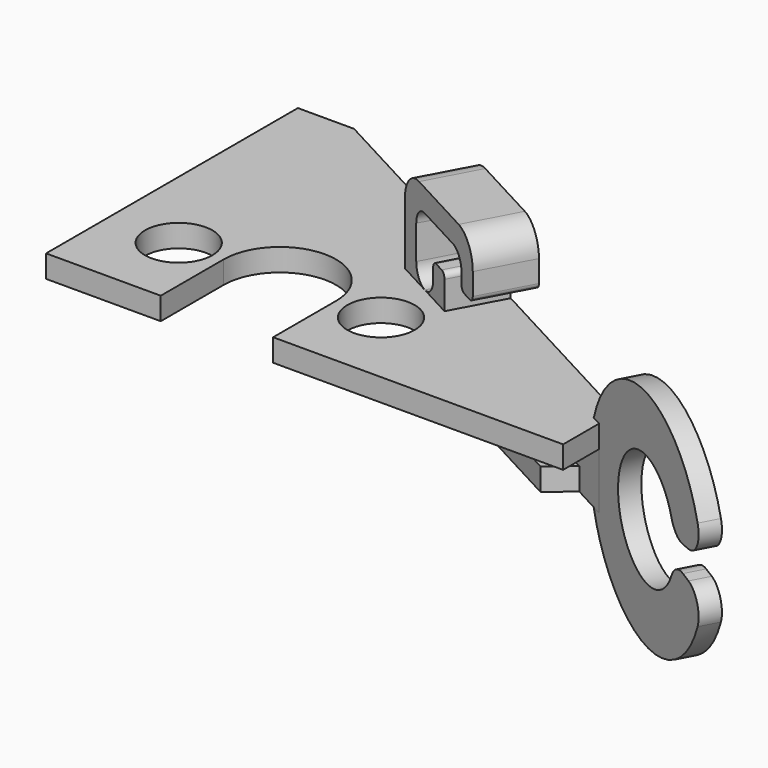
from build123d import *

# Parameters (mm, degrees)
F1_DEPTH  = 2
F2_R      = 3
F3_DEPTH  = 2
F4_W      = 2
F4_H      = 3
F5_DEPTH  = 5
F6_R      = 2.5
F7_R      = 1.49999
F8_R      = 0.5
F10_DEPTH = 5
F12_DEPTH = 2
F13_R     = 9.9401429079
F13_R_2   = 5
F14_DEPTH = 1.7623205361
F16_DEPTH = 1.7623205361
F17_R     = 2


# Not quite as in the source:
# - a fillet or chamfer is up to 0.001 mm smaller than in the source, because OpenCascade refuses the exact size


with BuildPart() as f1:
    # F0 (on Top) → F1 (new body)
    with BuildSketch(Plane.XY):
        Polygon((-19.7472184807, 28), (-19.7472184807, 0), (26.2527815193, 0), (26.2527815193, 6), (-14.7472184807, 28), align=None)
    extrude(amount=F1_DEPTH)

    # F2 (on face) → F3 (cut, through all)
    with BuildSketch(Plane.XY.offset(2)):
        with Locations((-13.5472184807, 7)):
            Circle(F2_R)
        with Locations((4.4527815193, 7)):
            Circle(F2_R)
        with BuildLine():
            Line((-9.5472184807, 7), (-9.5472184807, 0))
            Line((-9.5472184807, 0), (0.4527815193, 0))
            Line((0.4527815193, 0), (0.4527815193, 7))
            ThreePointArc((0.4527815193, 7), (-4.5472184807, 12), (-9.5472184807, 7))
        make_face()
    extrude(amount=-F3_DEPTH, mode=Mode.SUBTRACT)

    # F4 (on face) → F5 (join)
    with BuildSketch(Plane(origin=(8.3687511572, 15.5963089748, 0), x_dir=(-0.8811602681, 0.4728177048, 0), z_dir=(0.4728177048, 0.8811602681, 0))):
        Polygon((3.5210567079, 2), (5.5210567079, 2), (5.5210567079, 10), (-6.4789432921, 10), (-6.4789432921, 5.0490344875), (-4.4789432921, 5.0490344875), (-4.4789432921, 8), (3.5210567079, 8), align=None)
        with Locations((-0.4789432921, 3.5)):
            Rectangle(F4_W, F4_H)
    extrude(amount=-F5_DEPTH)

    # F6
    f6_edges = [f1.edges().sort_by_distance(p)[0] for p in [
        (12.895694, 10.330049, 10),
        (2.321771, 16.003862, 10),
    ]]
    fillet(f6_edges, radius=F6_R)

    # F7 (radius 1.5 in the source; OpenCascade refuses exactly that, so slightly less here)
    f7_edges = [f1.edges().sort_by_distance(p)[0] for p in [
        (6.727572, 13.639773, 2),
        (4.084092, 15.058226, 2),
        (11.133374, 11.275685, 8),
        (4.084092, 15.058226, 8),
    ]]
    fillet(f7_edges, radius=F7_R)

    # F8
    f8_edges = [f1.edges().sort_by_distance(p)[0] for p in [
        (12.895694, 10.330049, 5.049034),
        (11.133374, 11.275685, 5.049034),
        (8.489893, 12.694138, 5),
        (6.727572, 13.639773, 5),
    ]]
    fillet(f8_edges, radius=F8_R)

    # F9 (on face) → F10 (join)
    with BuildSketch(Plane(origin=(0, 0, 0), x_dir=(1, 0, 0), z_dir=(0, 0, -1))):
        Polygon((-19.7472184807, -26), (-19.7472184807, -28), (-14.7472184807, -28), (26.2527815193, -6), (26.2527815193, -4), (-14.7472184807, -26), align=None)
    extrude(amount=F10_DEPTH)

    # F11 (on face) → F12 (join)
    with BuildSketch(Plane(origin=(0, 0, -5), x_dir=(1, 0, 0), z_dir=(0, 0, -1))):
        Polygon((-15.9292627427, -23.7970993298), (-14.7472184807, -26), (1.1136663445, -17.4892813133), (-4.4741792579, -17.6504691673), align=None)
        Polygon((8.6295761581, -13.4563540963), (23.1687205811, -5.6548619669), (21.105516051, -3.9247790015), (8.7692722981, -10.5442268689), align=None)
    extrude(amount=-F12_DEPTH)

    # F13 (on face) → F14 (join, through all)
    with BuildSketch(Plane(origin=(8.3687511572, 15.5963089748, 0), x_dir=(-0.8811602681, 0.4728177048, 0), z_dir=(0.4728177048, 0.8811602681, 0))):
        with Locations((-29.5995731847, -1.5)):
            Circle(F13_R)
        with Locations((-29.5995731847, -1.5)):
            Circle(F13_R_2, mode=Mode.SUBTRACT)
    extrude(amount=-F14_DEPTH)

    # F15 (on face) → F16 (cut, through all)
    with BuildSketch(Plane(origin=(8.3687511572, 15.5963089748, 0), x_dir=(-0.8811602681, 0.4728177048, 0), z_dir=(0.4728177048, 0.8811602681, 0))):
        with BuildLine():
            ThreePointArc((-34.5031041583, -2.4774374616), (-34.5995731847, -1.5), (-34.5031041583, -0.5225625384))
            Line((-34.5031041583, -0.5225625384), (-39.4258868897, 0))
            ThreePointArc((-39.4258868897, 0), (-39.5397160926, -1.5), (-39.4258868897, -3))
            Line((-39.4258868897, -3), (-34.5031041583, -2.4774374616))
        make_face()
    extrude(amount=-F16_DEPTH, mode=Mode.SUBTRACT)

    # F17
    f17_edges = [f1.edges().sort_by_distance(p)[0] for p in [
        (42.692648, -3.821392, -3),
        (42.692648, -3.821392, 0),
        (38.354887, -1.493813, -0.522563),
        (38.354887, -1.493813, -2.477437),
    ]]
    fillet(f17_edges, radius=F17_R)


solid = f1.part
